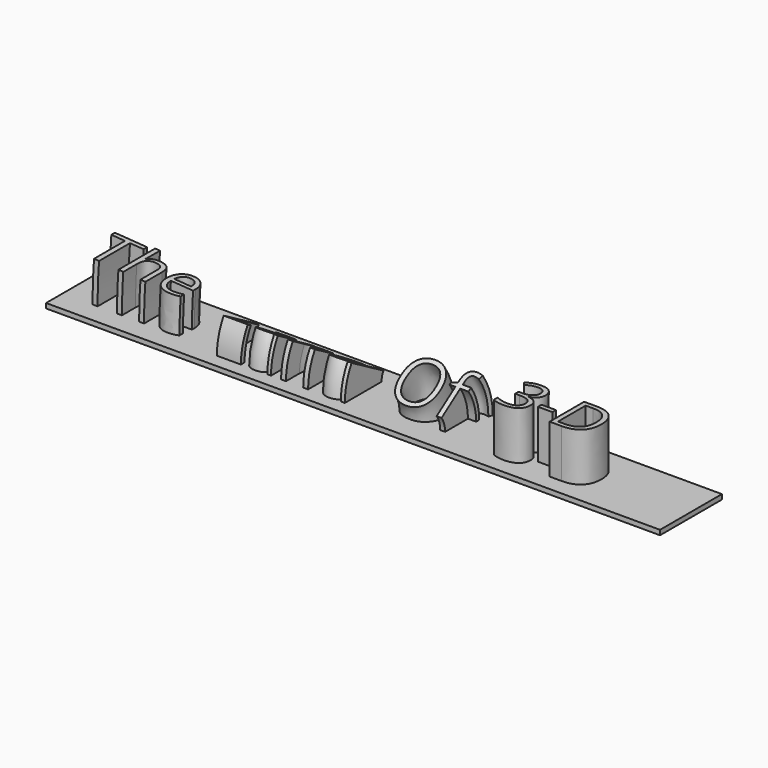
from build123d import *

# Parameters (mm, degrees)
F0_W         = 127
F0_H         = 16
F1_DEPTH     = 1
F5_TEXT_SIZE = 12.5
F6_DEPTH     = 10
F4_TEXT_SIZE = 12.5
F7_ANGLE     = 35
F2_TEXT_SIZE = 12.5
F8_ANGLE     = 4
F3_TEXT_SIZE = 12.5
F9_ANGLE     = 30


# Not quite as in the source:
# - Text() gives the source's letters only with a copy of the font that has no kerning and outlines rounded to 1/6400 em; it was checked with that copy


with BuildPart() as f1:
    # F0 (on Top) → F1 (new body)
    with BuildSketch(Plane.XY):
        Rectangle(F0_W, F0_H)
    extrude(amount=F1_DEPTH)

    # F5 (on face) → F6 (join)
    with BuildSketch(Plane.XY.offset(1)):
        with Locations((25.5465835604, -4.6034566966)):
            Text('3-D', F5_TEXT_SIZE, font='Open Sans', text_align=(TextAlign.LEFT, TextAlign.BOTTOM))
    extrude(amount=F6_DEPTH)

    # F4 (on face) → F7 (revolve)
    with BuildSketch(Plane.XY.offset(1)):
        with Locations((2.8665268328, -2.9364474267)):
            Text('Of', F4_TEXT_SIZE, font='Open Sans', text_align=(TextAlign.LEFT, TextAlign.BOTTOM))
    revolve(axis=Axis((0, -8, 1), (1, 0, 0)), revolution_arc=F7_ANGLE)

    # F2 (on face) → F8 (revolve)
    with BuildSketch(Plane.XY.offset(1)):
        with Locations((-60.240726671, -3.7139668971)):
            Text('The', F2_TEXT_SIZE, font='Open Sans', text_align=(TextAlign.LEFT, TextAlign.BOTTOM))
    revolve(axis=Axis((63.5, 0, 1), (0, 1, 0)), revolution_arc=F8_ANGLE)

    # F3 (on face) → F9 (revolve)
    with BuildSketch(Plane.XY.offset(1)):
        with Locations((-31.6739654026, -5.160415596)):
            Text('Land', F3_TEXT_SIZE, font='Open Sans', text_align=(TextAlign.LEFT, TextAlign.BOTTOM))
    revolve(axis=Axis((0, 8, 1), (-1, 0, 0)), revolution_arc=F9_ANGLE)


solid = f1.part
